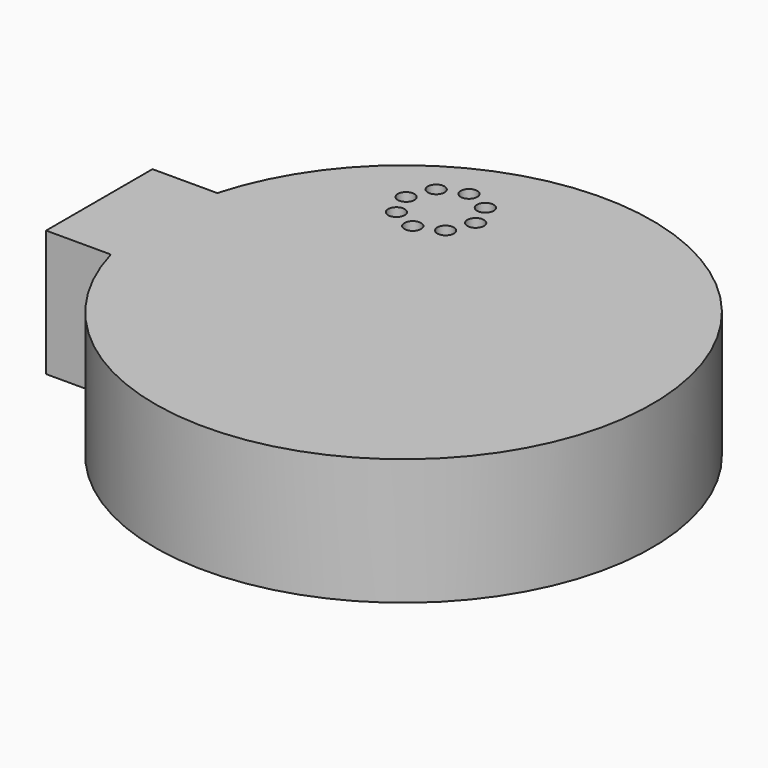
from build123d import *

# Parameters (mm, degrees)
F0_W             = 1
F0_H             = 20
F1_DEPTH         = 19
F2_W             = 50
F2_H             = 18.5
F3_DEPTH         = 17.2
F4_W             = 46
F4_H             = 18.5
F5_DEPTH         = 0.5
F7_DEPTH         = 11
F10_DEPTH        = 5
F8_R             = 7
F11_DEPTH        = 15
F12_R            = 1.25
F13_DEPTH        = 4
F13_COPIES_COUNT = 8


# Not quite as in the source:
# - a pattern or mirror of a feature is missing from the dataset's text; its kind, count and spacing are read off the source's solid


with BuildPart() as f1:
    # F0 (on Top) → F1 (new body)
    with BuildSketch(Plane.XY):
        with BuildLine():
            ThreePointArc((-36.0123676672, -10), (5.0462056754, -37.0327751226), (37.375, 0))
            ThreePointArc((37.375, 0), (5.0462056754, 37.0327751226), (-36.0123676672, 10))
            Line((-36.0123676672, 10), (-30, 10))
            Line((-30, 10), (-30, -10))
            Line((-30, -10), (-36.0123676672, -10))
        make_face()
        with BuildLine():
            Line((-30, 10), (-36.0123676672, 10))
            ThreePointArc((-36.0123676672, 10), (-37.375, 0), (-36.0123676672, -10))
            Line((-36.0123676672, -10), (-30, -10))
            Line((-30, -10), (-30, 10))
        make_face()
        with BuildLine():
            ThreePointArc((-36.0123676672, -10), (-37.375, 0), (-36.0123676672, 10))
            Line((-36.0123676672, 10), (-44.75, 10))
            Line((-44.75, 10), (-44.75, -10))
            Line((-44.75, -10), (-36.0123676672, -10))
        make_face()
        with Locations((-45.25, 0)):
            Rectangle(F0_W, F0_H)
    extrude(amount=F1_DEPTH)

    # F2 (on face) → F3 (cut)
    with BuildSketch(Plane(origin=(0, 0, 0), x_dir=(1, 0, 0), z_dir=(0, 0, -1))):
        with Locations((-20.75, 0)):
            Rectangle(F2_W, F2_H)
    extrude(amount=-F3_DEPTH, mode=Mode.SUBTRACT)

    # F4 (on face) → F5 (cut)
    with BuildSketch(Plane(origin=(0, 0, 17.2), x_dir=(1, 0, 0), z_dir=(0, 0, -1))):
        with Locations((-20.75, 0)):
            Rectangle(F4_W, F4_H)
    extrude(amount=-F5_DEPTH, mode=Mode.SUBTRACT)

    # F6 (on face) → F7 (cut)
    with BuildSketch(Plane(origin=(0, 0, 0), x_dir=(1, 0, 0), z_dir=(0, 0, -1))):
        Polygon((30.5, 20.4567786688), (4.25, 20.4567786688), (4.25, 9.25), (4.25, -9.25), (4.25, -19.5432213312), (30.5, -19.5432213312), align=None)
    extrude(amount=-F7_DEPTH, mode=Mode.SUBTRACT)

    # F9 (on face) → F10 (cut)
    with BuildSketch(Plane(origin=(0, 0, 0), x_dir=(1, 0, 0), z_dir=(0, 0, -1))):
        Polygon((-27.0342712475, -9.25), (-12.8921356237, -23.3921356237), (1.25, -9.25), align=None)
    extrude(amount=-F10_DEPTH, mode=Mode.SUBTRACT)

    # F8 (on face) → F11 (cut)
    with BuildSketch(Plane(origin=(0, 0, 0), x_dir=(1, 0, 0), z_dir=(0, 0, -1))):
        with Locations((-12.8315193579, -23.0468716472)):
            Circle(F8_R)
    extrude(amount=-F11_DEPTH, mode=Mode.SUBTRACT)

    # F12 (on face) → F13 (cut)
    with BuildSketch(Plane(origin=(0, 0, 15), x_dir=(1, 0, 0), z_dir=(0, 0, -1))):
        with Locations((-12.8591003243, -17.7969360865)):
            Circle(F12_R)
    f13 = extrude(amount=-F13_DEPTH, mode=Mode.SUBTRACT)

    # F13_copies: F13 ×8 about axis
    f13_copies_axis = Axis((-12.831519, 23.046872, 0), (0, 0, 1))
    for i in range(1, F13_COPIES_COUNT):
        add(f13.rotate(f13_copies_axis, i * 360 / F13_COPIES_COUNT), mode=Mode.SUBTRACT)


solid = f1.part
